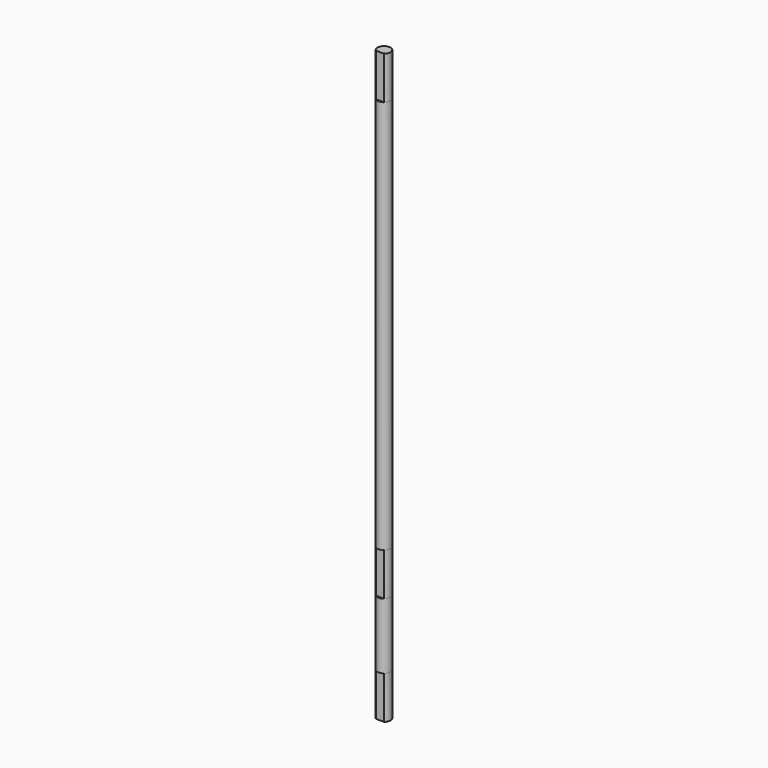
from build123d import *
from build123d import SkipClean  # not in build123d's __all__

# Parameters (mm, degrees)
F0_R     = 2.5
F1_DEPTH = 152.4
F3_DEPTH = 16.5250114
F5_DEPTH = 16.5250114
F6_R     = 2.5
F7_DEPTH = 25.4
F9_DEPTH = 16.5250114


# Not quite as in the source:
# - after a boolean that leaves OpenCascade's solid faulty, fix() repairs it


with BuildPart() as f1:
    # F0 (on Top) → F1 (new body)
    with BuildSketch(Plane.XY):
        Circle(F0_R)
    extrude(amount=F1_DEPTH)

    # F2 (on face) → F3 (join)
    with BuildSketch(Plane.XY.offset(152.4)):
        with BuildLine():
            Line((0, -1.9312803396), (1.5875, -1.9312803396))
            ThreePointArc((1.5875, -1.9312803396), (0, 2.5), (-1.5875, -1.9312803396))
            Line((-1.5875, -1.9312803396), (0, -1.9312803396))
        make_face()
    extrude(amount=F3_DEPTH)

    # F4 (on face) → F5 (join)
    with BuildSketch(Plane(origin=(0, 0, 0), x_dir=(1, 0, 0), z_dir=(0, 0, -1))):
        with BuildLine():
            Line((1.5875, 1.9312803396), (-1.5875, 1.9312803396))
            ThreePointArc((-1.5875, 1.9312803396), (0, -2.5), (1.5875, 1.9312803396))
        make_face()
    with SkipClean():  # cleaning this boolean's faces spoils the solid; the shape is the same uncleaned
        extrude(amount=F5_DEPTH)

    # F6 (on face) → F7 (join)
    with BuildSketch(Plane(origin=(0, 0, -16.5250114), x_dir=(1, 0, 0), z_dir=(0, 0, -1))):
        Circle(F6_R)
    extrude(amount=F7_DEPTH)

    add(f1.part.fix(), mode=Mode.REPLACE)

    # F8 (on face) → F9 (join)
    with BuildSketch(Plane(origin=(0, 0, -41.9250114), x_dir=(1, 0, 0), z_dir=(0, 0, -1))):
        with BuildLine():
            Line((1.5875, 1.9312803396), (-1.5875, 1.9312803396))
            ThreePointArc((-1.5875, 1.9312803396), (0, -2.5), (1.5875, 1.9312803396))
        make_face()
    extrude(amount=F9_DEPTH)


solid = f1.part
